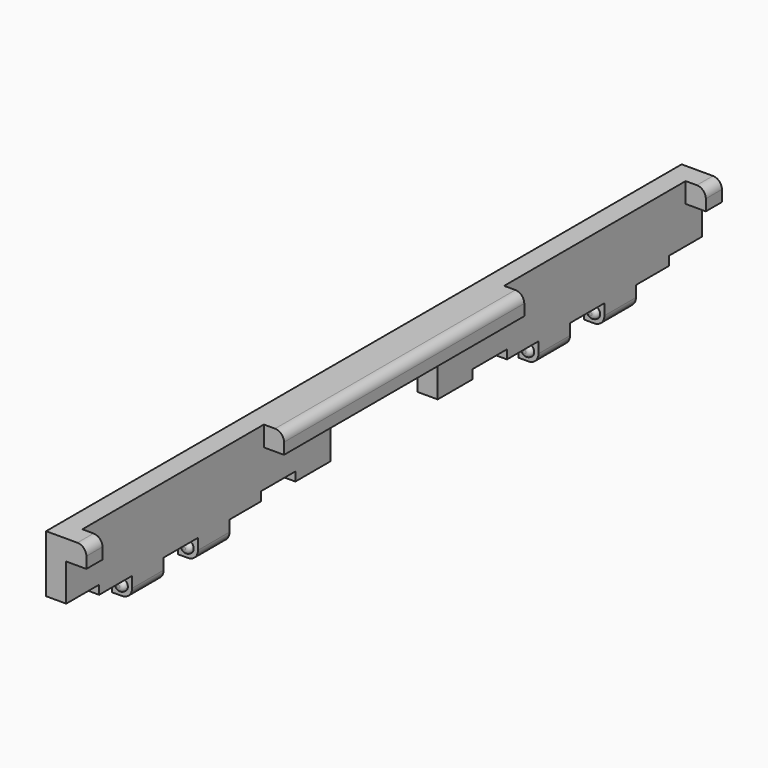
from build123d import *

# Parameters (mm, degrees)
F0_R      = 1.5
F1_DEPTH  = 159.1
F2_DEPTH  = 150.3
F3_DEPTH  = 177.5
F4_DEPTH  = 140.7
F5_DEPTH  = 131.9
F6_DEPTH  = 45.6
F7_DEPTH  = 36.8
F8_DEPTH  = 27.2
F9_DEPTH  = 18.4
F10_DEPTH = 173
F11_DEPTH = 122.3
F12_DEPTH = 55.2
F13_DEPTH = 4.5
F14_W     = 30
F14_H     = 7
F14_W_2   = 9.6
F14_H_2   = 2
F14_W_3   = 9.2
F15_DEPTH = 25
F16_R     = 1.5
F16_R_2   = 1.3
F17_R     = 1.5
F17_R_2   = 1.3
F18_R     = 1.5
F18_R_2   = 1.3
F19_R     = 1.5
F19_R_2   = 1.3
F20_DEPTH = 8.8
F21_DEPTH = 9.8
F22_DEPTH = 2
F23_R     = 0.99999


# Not quite as in the source:
# - a fillet or chamfer is up to 0.001 mm smaller than in the source, because OpenCascade refuses the exact size
# - a feature names something its author has since deleted; it is built from what else it names


with BuildPart() as f1:
    # F0 (on Front) → F1 (new body)
    with BuildSketch(Plane.XZ):
        with BuildLine():
            Line((-0.0833333333, -31.4652777778), (-0.0833333333, -29.0152777778))
            Line((-0.0833333333, -29.0152777778), (-4.5833333333, -29.0152777778))
            Line((-4.5833333333, -29.0152777778), (-4.5833333333, -31.4652777778))
            Line((-4.5833333333, -31.4652777778), (-4.5833333333, -33.7152777778))
            Line((-4.5833333333, -33.7152777778), (-2.3333333333, -33.7152777778))
            ThreePointArc((-2.3333333333, -33.7152777778), (-0.7423430757, -33.0562680354), (-0.0833333333, -31.4652777778))
        make_face()
        with Locations((-2.3333333333, -31.4652777778)):
            Circle(F0_R, mode=Mode.SUBTRACT)
        Polygon((-0.0833333333, -29.0152777778), (-0.0833333333, -18.7152777778), (-0.0833333333, -14.2152777778), (-4.5833333333, -14.2152777778), (-4.5833333333, -29.0152777778), align=None)
    extrude(amount=F1_DEPTH)

    # F0 (on Front) → F2 (cut)
    with BuildSketch(Plane.XZ):
        with BuildLine():
            Line((-0.0833333333, -14.2152777778), (-0.0833333333, -18.7152777778))
            Line((-0.0833333333, -18.7152777778), (4.4166666667, -18.7152777778))
            Line((4.4166666667, -18.7152777778), (4.4166666667, -16.2152777778))
            ThreePointArc((4.4166666667, -16.2152777778), (3.830880229, -14.8010642154), (2.4166666667, -14.2152777778))
            Line((2.4166666667, -14.2152777778), (-0.0833333333, -14.2152777778))
        make_face()
        with BuildLine():
            Line((-0.0833333333, -31.4652777778), (-0.0833333333, -29.0152777778))
            Line((-0.0833333333, -29.0152777778), (-4.5833333333, -29.0152777778))
            Line((-4.5833333333, -29.0152777778), (-4.5833333333, -31.4652777778))
            Line((-4.5833333333, -31.4652777778), (-4.5833333333, -33.7152777778))
            Line((-4.5833333333, -33.7152777778), (-2.3333333333, -33.7152777778))
            ThreePointArc((-2.3333333333, -33.7152777778), (-0.7423430757, -33.0562680354), (-0.0833333333, -31.4652777778))
        make_face()
        with Locations((-2.3333333333, -31.4652777778)):
            Circle(F0_R, mode=Mode.SUBTRACT)
    extrude(amount=F2_DEPTH, mode=Mode.SUBTRACT)

    # F0 (on Front) → F3 (join)
    with BuildSketch(Plane.XZ):
        with BuildLine():
            Line((-0.0833333333, -14.2152777778), (-0.0833333333, -18.7152777778))
            Line((-0.0833333333, -18.7152777778), (4.4166666667, -18.7152777778))
            Line((4.4166666667, -18.7152777778), (4.4166666667, -16.2152777778))
            ThreePointArc((4.4166666667, -16.2152777778), (3.830880229, -14.8010642154), (2.4166666667, -14.2152777778))
            Line((2.4166666667, -14.2152777778), (-0.0833333333, -14.2152777778))
        make_face()
        Polygon((-0.0833333333, -29.0152777778), (-0.0833333333, -18.7152777778), (-0.0833333333, -14.2152777778), (-4.5833333333, -14.2152777778), (-4.5833333333, -29.0152777778), align=None)
    extrude(amount=F3_DEPTH)

    # F0 (on Front) → F4 (join)
    with BuildSketch(Plane.XZ):
        with BuildLine():
            Line((-0.0833333333, -31.4652777778), (-0.0833333333, -29.0152777778))
            Line((-0.0833333333, -29.0152777778), (-4.5833333333, -29.0152777778))
            Line((-4.5833333333, -29.0152777778), (-4.5833333333, -31.4652777778))
            Line((-4.5833333333, -31.4652777778), (-4.5833333333, -33.7152777778))
            Line((-4.5833333333, -33.7152777778), (-2.3333333333, -33.7152777778))
            ThreePointArc((-2.3333333333, -33.7152777778), (-0.7423430757, -33.0562680354), (-0.0833333333, -31.4652777778))
        make_face()
        with Locations((-2.3333333333, -31.4652777778)):
            Circle(F0_R, mode=Mode.SUBTRACT)
    extrude(amount=F4_DEPTH)

    # F0 (on Front) → F5 (cut)
    with BuildSketch(Plane.XZ):
        with BuildLine():
            Line((-0.0833333333, -31.4652777778), (-0.0833333333, -29.0152777778))
            Line((-0.0833333333, -29.0152777778), (-4.5833333333, -29.0152777778))
            Line((-4.5833333333, -29.0152777778), (-4.5833333333, -31.4652777778))
            Line((-4.5833333333, -31.4652777778), (-4.5833333333, -33.7152777778))
            Line((-4.5833333333, -33.7152777778), (-2.3333333333, -33.7152777778))
            ThreePointArc((-2.3333333333, -33.7152777778), (-0.7423430757, -33.0562680354), (-0.0833333333, -31.4652777778))
        make_face()
        with Locations((-2.3333333333, -31.4652777778)):
            Circle(F0_R, mode=Mode.SUBTRACT)
    extrude(amount=F5_DEPTH, mode=Mode.SUBTRACT)

    # F0 (on Front) → F6 (join)
    with BuildSketch(Plane.XZ):
        with BuildLine():
            Line((-0.0833333333, -31.4652777778), (-0.0833333333, -29.0152777778))
            Line((-0.0833333333, -29.0152777778), (-4.5833333333, -29.0152777778))
            Line((-4.5833333333, -29.0152777778), (-4.5833333333, -31.4652777778))
            Line((-4.5833333333, -31.4652777778), (-4.5833333333, -33.7152777778))
            Line((-4.5833333333, -33.7152777778), (-2.3333333333, -33.7152777778))
            ThreePointArc((-2.3333333333, -33.7152777778), (-0.7423430757, -33.0562680354), (-0.0833333333, -31.4652777778))
        make_face()
        with Locations((-2.3333333333, -31.4652777778)):
            Circle(F0_R, mode=Mode.SUBTRACT)
    extrude(amount=F6_DEPTH)

    # F0 (on Front) → F7 (cut)
    with BuildSketch(Plane.XZ):
        with BuildLine():
            Line((-0.0833333333, -31.4652777778), (-0.0833333333, -29.0152777778))
            Line((-0.0833333333, -29.0152777778), (-4.5833333333, -29.0152777778))
            Line((-4.5833333333, -29.0152777778), (-4.5833333333, -31.4652777778))
            Line((-4.5833333333, -31.4652777778), (-4.5833333333, -33.7152777778))
            Line((-4.5833333333, -33.7152777778), (-2.3333333333, -33.7152777778))
            ThreePointArc((-2.3333333333, -33.7152777778), (-0.7423430757, -33.0562680354), (-0.0833333333, -31.4652777778))
        make_face()
        with Locations((-2.3333333333, -31.4652777778)):
            Circle(F0_R, mode=Mode.SUBTRACT)
    extrude(amount=F7_DEPTH, mode=Mode.SUBTRACT)

    # F0 (on Front) → F8 (join)
    with BuildSketch(Plane.XZ):
        with BuildLine():
            Line((-0.0833333333, -31.4652777778), (-0.0833333333, -29.0152777778))
            Line((-0.0833333333, -29.0152777778), (-4.5833333333, -29.0152777778))
            Line((-4.5833333333, -29.0152777778), (-4.5833333333, -31.4652777778))
            Line((-4.5833333333, -31.4652777778), (-4.5833333333, -33.7152777778))
            Line((-4.5833333333, -33.7152777778), (-2.3333333333, -33.7152777778))
            ThreePointArc((-2.3333333333, -33.7152777778), (-0.7423430757, -33.0562680354), (-0.0833333333, -31.4652777778))
        make_face()
        with Locations((-2.3333333333, -31.4652777778)):
            Circle(F0_R, mode=Mode.SUBTRACT)
    extrude(amount=F8_DEPTH)

    # F0 (on Front) → F9 (cut)
    with BuildSketch(Plane.XZ):
        with BuildLine():
            Line((-0.0833333333, -31.4652777778), (-0.0833333333, -29.0152777778))
            Line((-0.0833333333, -29.0152777778), (-4.5833333333, -29.0152777778))
            Line((-4.5833333333, -29.0152777778), (-4.5833333333, -31.4652777778))
            Line((-4.5833333333, -31.4652777778), (-4.5833333333, -33.7152777778))
            Line((-4.5833333333, -33.7152777778), (-2.3333333333, -33.7152777778))
            ThreePointArc((-2.3333333333, -33.7152777778), (-0.7423430757, -33.0562680354), (-0.0833333333, -31.4652777778))
        make_face()
        with Locations((-2.3333333333, -31.4652777778)):
            Circle(F0_R, mode=Mode.SUBTRACT)
    extrude(amount=F9_DEPTH, mode=Mode.SUBTRACT)

    # F0 (on Front) → F10 (cut)
    with BuildSketch(Plane.XZ):
        with BuildLine():
            Line((-0.0833333333, -14.2152777778), (-0.0833333333, -18.7152777778))
            Line((-0.0833333333, -18.7152777778), (4.4166666667, -18.7152777778))
            Line((4.4166666667, -18.7152777778), (4.4166666667, -16.2152777778))
            ThreePointArc((4.4166666667, -16.2152777778), (3.830880229, -14.8010642154), (2.4166666667, -14.2152777778))
            Line((2.4166666667, -14.2152777778), (-0.0833333333, -14.2152777778))
        make_face()
    extrude(amount=F10_DEPTH, mode=Mode.SUBTRACT)

    # F0 (on Front) → F11 (join)
    with BuildSketch(Plane.XZ):
        with BuildLine():
            Line((-0.0833333333, -14.2152777778), (-0.0833333333, -18.7152777778))
            Line((-0.0833333333, -18.7152777778), (4.4166666667, -18.7152777778))
            Line((4.4166666667, -18.7152777778), (4.4166666667, -16.2152777778))
            ThreePointArc((4.4166666667, -16.2152777778), (3.830880229, -14.8010642154), (2.4166666667, -14.2152777778))
            Line((2.4166666667, -14.2152777778), (-0.0833333333, -14.2152777778))
        make_face()
    extrude(amount=F11_DEPTH)

    # F0 (on Front) → F12 (cut)
    with BuildSketch(Plane.XZ):
        with BuildLine():
            Line((-0.0833333333, -14.2152777778), (-0.0833333333, -18.7152777778))
            Line((-0.0833333333, -18.7152777778), (4.4166666667, -18.7152777778))
            Line((4.4166666667, -18.7152777778), (4.4166666667, -16.2152777778))
            ThreePointArc((4.4166666667, -16.2152777778), (3.830880229, -14.8010642154), (2.4166666667, -14.2152777778))
            Line((2.4166666667, -14.2152777778), (-0.0833333333, -14.2152777778))
        make_face()
    extrude(amount=F12_DEPTH, mode=Mode.SUBTRACT)

    # F0 (on Front) → F13 (join)
    with BuildSketch(Plane.XZ):
        with BuildLine():
            Line((-0.0833333333, -14.2152777778), (-0.0833333333, -18.7152777778))
            Line((-0.0833333333, -18.7152777778), (4.4166666667, -18.7152777778))
            Line((4.4166666667, -18.7152777778), (4.4166666667, -16.2152777778))
            ThreePointArc((4.4166666667, -16.2152777778), (3.830880229, -14.8010642154), (2.4166666667, -14.2152777778))
            Line((2.4166666667, -14.2152777778), (-0.0833333333, -14.2152777778))
        make_face()
    extrude(amount=F13_DEPTH)

    # F14 (on face) → F15 (cut)
    with BuildSketch(Plane.YZ.offset(-0.0833333333)):
        with Locations((-88.75, -25.5152777778)):
            Rectangle(F14_W, F14_H)
        with Locations((-59.2, -28.0152777778)):
            Rectangle(F14_W_2, F14_H_2)
        with Locations((-4.6, -28.0152777778)):
            Rectangle(F14_W_3, F14_H_2)
        with Locations((-118.3, -28.0152777778)):
            Rectangle(F14_W_2, F14_H_2)
        with Locations((-172.9, -28.0152777778)):
            Rectangle(F14_W_3, F14_H_2)
    extrude(amount=-F15_DEPTH, mode=Mode.SUBTRACT)

    # F16 (on face) + F17 (on face) + F18 (on face) + F19 (on face) → F20 (join)
    with BuildSketch(Plane(origin=(0, -18.4, 0), x_dir=(-1, 0, 0), z_dir=(0, 1, 0))):
        with Locations((2.3333333333, -31.4652777778)):
            Circle(F16_R)
        with Locations((2.3333333333, -31.4652777778)):
            Circle(F16_R_2, mode=Mode.SUBTRACT)
    with BuildSketch(Plane(origin=(0, -36.8, 0), x_dir=(-1, 0, 0), z_dir=(0, 1, 0))):
        with Locations((2.3333333333, -31.4652777778)):
            Circle(F17_R)
        with Locations((2.3333333333, -31.4652777778)):
            Circle(F17_R_2, mode=Mode.SUBTRACT)
    with BuildSketch(Plane(origin=(0, -131.9, 0), x_dir=(-1, 0, 0), z_dir=(0, 1, 0))):
        with Locations((2.3333333333, -31.4652777778)):
            Circle(F18_R)
        with Locations((2.3333333333, -31.4652777778)):
            Circle(F18_R_2, mode=Mode.SUBTRACT)
    with BuildSketch(Plane(origin=(0, -150.3, 0), x_dir=(-1, 0, 0), z_dir=(0, 1, 0))):
        with Locations((2.3333333333, -31.4652777778)):
            Circle(F19_R)
        with Locations((2.3333333333, -31.4652777778)):
            Circle(F19_R_2, mode=Mode.SUBTRACT)
    extrude(amount=-F20_DEPTH)

    # F16 (on face) + F17 (on face) + F18 (on face) + F19 (on face) → F21 (join)
    with BuildSketch(Plane(origin=(0, -18.4, 0), x_dir=(-1, 0, 0), z_dir=(0, 1, 0))):
        with Locations((2.3333333333, -31.4652777778)):
            Circle(F16_R_2)
    with BuildSketch(Plane(origin=(0, -36.8, 0), x_dir=(-1, 0, 0), z_dir=(0, 1, 0))):
        with Locations((2.3333333333, -31.4652777778)):
            Circle(F17_R_2)
    with BuildSketch(Plane(origin=(0, -131.9, 0), x_dir=(-1, 0, 0), z_dir=(0, 1, 0))):
        with Locations((2.3333333333, -31.4652777778)):
            Circle(F18_R_2)
    with BuildSketch(Plane(origin=(0, -150.3, 0), x_dir=(-1, 0, 0), z_dir=(0, 1, 0))):
        with Locations((2.3333333333, -31.4652777778)):
            Circle(F19_R_2)
    extrude(amount=-F21_DEPTH)

    # F16 (on face) + F17 (on face) + F18 (on face) + F19 (on face) → F22 (cut)
    with BuildSketch(Plane(origin=(0, -18.4, 0), x_dir=(-1, 0, 0), z_dir=(0, 1, 0))):
        with Locations((2.3333333333, -31.4652777778)):
            Circle(F16_R)
        with Locations((2.3333333333, -31.4652777778)):
            Circle(F16_R_2, mode=Mode.SUBTRACT)
        with Locations((2.3333333333, -31.4652777778)):
            Circle(F16_R_2)
    with BuildSketch(Plane(origin=(0, -36.8, 0), x_dir=(-1, 0, 0), z_dir=(0, 1, 0))):
        with Locations((2.3333333333, -31.4652777778)):
            Circle(F17_R)
        with Locations((2.3333333333, -31.4652777778)):
            Circle(F17_R_2, mode=Mode.SUBTRACT)
        with Locations((2.3333333333, -31.4652777778)):
            Circle(F17_R_2)
    with BuildSketch(Plane(origin=(0, -131.9, 0), x_dir=(-1, 0, 0), z_dir=(0, 1, 0))):
        with Locations((2.3333333333, -31.4652777778)):
            Circle(F18_R)
        with Locations((2.3333333333, -31.4652777778)):
            Circle(F18_R_2, mode=Mode.SUBTRACT)
        with Locations((2.3333333333, -31.4652777778)):
            Circle(F18_R_2)
    with BuildSketch(Plane(origin=(0, -150.3, 0), x_dir=(-1, 0, 0), z_dir=(0, 1, 0))):
        with Locations((2.3333333333, -31.4652777778)):
            Circle(F19_R)
        with Locations((2.3333333333, -31.4652777778)):
            Circle(F19_R_2, mode=Mode.SUBTRACT)
        with Locations((2.3333333333, -31.4652777778)):
            Circle(F19_R_2)
    extrude(amount=-F22_DEPTH, mode=Mode.SUBTRACT)

    # F23 (radius 1 in the source; OpenCascade refuses exactly that, so slightly less here)
    f23_edges = [f1.edges().sort_by_distance(p)[0] for p in [
        (-1.033333, -28.2, -31.465278),
        (-1.033333, -46.6, -31.465278),
        (-1.033333, -141.7, -31.465278),
        (-1.033333, -160.1, -31.465278),
    ]]
    fillet(f23_edges, radius=F23_R)


solid = f1.part
